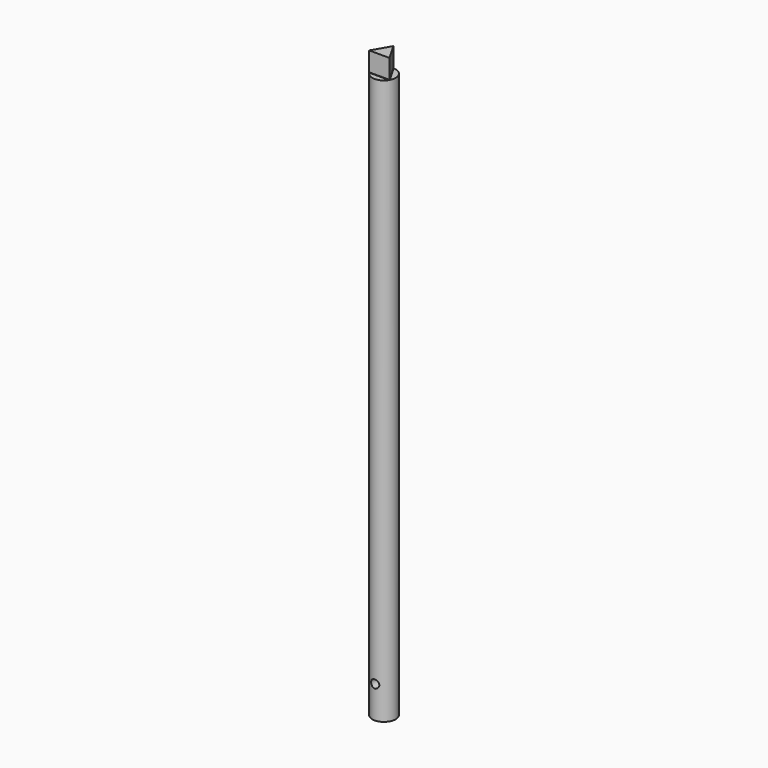
from build123d import *

# Parameters (mm, degrees)
F0_R        = 6
F1_DEPTH    = 300
F2_R        = 11
F3_DEPTH    = 10
F4_T4_DEPTH = 11.3923048454
F4_S5_R     = 6
F4_T6_DEPTH = 7
F5_T4_DEPTH = 11.3923048454
F5_S5_R     = 6
F5_T6_DEPTH = 7
F6_R        = 0.2
F9_D        = 4.2


# Not quite as in the source:
# - a fillet or chamfer that OpenCascade refuses, or shapes differently, is made with other operations: its cross-section is extruded or revolved along the edge and cut away or added


with BuildPart() as f1:
    # F0 (on Top) → F1 (new body)
    with BuildSketch(Plane.XY):
        Circle(F0_R)
    extrude(amount=F1_DEPTH)

    # F2 (on face) → F3 (cut)
    with BuildSketch(Plane.XY.offset(300)):
        Circle(F2_R)
        Polygon((5.1961524227, -3), (-5.1961524227, -3), (0, 6), align=None, mode=Mode.SUBTRACT)
    extrude(amount=-F3_DEPTH, mode=Mode.SUBTRACT)

    # F4: fillet of radius 0.2 on 1 edges, made by hand


with BuildPart() as f4_tool2:
    # F4_s3 → F4_t4 (new body)
    with BuildSketch(Plane.YZ.offset(5.6961524227)):
        with BuildLine():
            ThreePointArc((-3.2, 290), (-3.0585786438, 290.0585786438), (-3, 290.2))
            Line((-3, 290.2), (-3, 290))
            Line((-3, 290), (-3.2, 290))
        make_face()
    extrude(amount=-F4_T4_DEPTH)

    # F4_s5 → F4_t6 (intersect, symmetric)
    with BuildSketch(Plane.XY.offset(290.1)):
        Circle(F4_S5_R)
    extrude(amount=F4_T6_DEPTH, both=True, mode=Mode.INTERSECT)

    split(bisect_by=Plane(origin=(2.5980762114, 1.5, 0), x_dir=(0, 0, 1), z_dir=(-0.8660254038, -0.5, 0)), keep=Keep.TOP)

    split(bisect_by=Plane(origin=(-2.5980762114, 1.5, 0), x_dir=(0, 0, 1), z_dir=(0.8660254038, -0.5, 0)), keep=Keep.TOP)


with BuildPart() as f1_1:
    add(f1.part)

    # F4_t1: union F4_tool2
    add(f4_tool2.part)

    # F5: fillet of radius 0.2 on 1 edges, made by hand


with BuildPart() as f5_tool2:
    # F5_s3 → F5_t4 (new body)
    with BuildSketch(Plane(origin=(-2.8480762114, -4.9330127019, 0), x_dir=(0, 0, 1), z_dir=(0.5, 0.8660254038, 0))):
        with BuildLine():
            ThreePointArc((290, -3.2), (290.0585786438, -3.0585786438), (290.2, -3))
            Line((290.2, -3), (290, -3))
            Line((290, -3), (290, -3.2))
        make_face()
    extrude(amount=F5_T4_DEPTH)

    # F5_s5 → F5_t6 (intersect, symmetric)
    with BuildSketch(Plane.XY.offset(290.1)):
        Circle(F5_S5_R)
    extrude(amount=F5_T6_DEPTH, both=True, mode=Mode.INTERSECT)

    split(bisect_by=Plane(origin=(2.5980762114, 1.5, 0), x_dir=(0, 0, 1), z_dir=(-0.8660254038, -0.5, 0)), keep=Keep.TOP)


with BuildPart() as f1_2:
    add(f1_1.part)

    # F5_t1: union F5_tool2
    add(f5_tool2.part)

    # F6
    f6_edges = [f1_2.edges().sort_by_distance(p)[0] for p in [
        (2.598076, 1.5, 290),
    ]]
    fillet(f6_edges, radius=F6_R)

    # F9 (through all)
    with Locations(Plane.XZ.offset(6)):
        with Locations((0, 16.5)):
            Hole(F9_D / 2)


solid = f1_2.part
